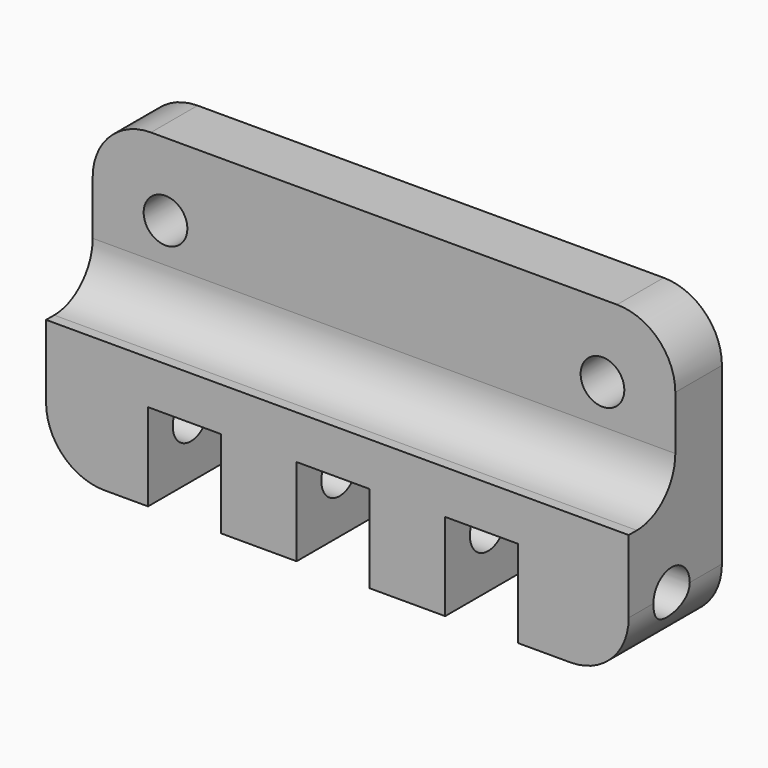
from build123d import *

# Parameters (mm, degrees)
F1_DEPTH    = 127
F2_R        = 4.7625
F3_DEPTH    = 25.4
F4_W        = 15.875
F4_H        = 19.05
F5_DEPTH    = 25.401
F6_R        = 4.953
F7_DEPTH    = 127.001
F8_T1_DEPTH = 76.2
F8_T3_DEPTH = 88.9


# Not quite as in the source:
# - a fillet or chamfer that OpenCascade refuses, or shapes differently, is made with other operations: its cross-section is extruded or revolved along the edge and cut away or added


with BuildPart() as f1:
    # F0 (on Right) → F1 (new body)
    with BuildSketch(Plane.YZ):
        with BuildLine():
            Line((0, 28.575), (0, 0))
            Line((0, 0), (25.4, 0))
            Line((25.4, 0), (25.4, 63.5))
            Line((25.4, 63.5), (12.7, 63.5))
            Line((12.7, 63.5), (12.7, 39.0525))
            ThreePointArc((12.7, 39.0525), (9.6312112999, 31.6437887001), (2.2225, 28.575))
            Line((2.2225, 28.575), (0, 28.575))
        make_face()
    extrude(amount=F1_DEPTH)

    # F2 (on face) → F3 (cut)
    with BuildSketch(Plane.XZ.offset(-12.7)):
        with Locations((111.125, 47.625)):
            Circle(F2_R)
        with Locations((15.875, 47.625)):
            Circle(F2_R)
    extrude(amount=-F3_DEPTH, mode=Mode.SUBTRACT)

    # F4 (on face) → F5 (cut, through all)
    with BuildSketch(Plane.XZ):
        with Locations((94.9325, 9.525)):
            Rectangle(F4_W, F4_H)
        with Locations((62.5475, 9.525)):
            Rectangle(F4_W, F4_H)
        with Locations((30.1625, 9.525)):
            Rectangle(F4_W, F4_H)
    extrude(amount=-F5_DEPTH, mode=Mode.SUBTRACT)

    # F6 (on face) → F7 (cut, through all)
    with BuildSketch(Plane.YZ.offset(127)):
        with Locations((11.684, 12.7)):
            Circle(F6_R)
    extrude(amount=-F7_DEPTH, mode=Mode.SUBTRACT)

    # F8: fillet of radius 12.7 on 4 edges, made by hand

    # F8_s2 → F8_t1 (cut)
    with BuildSketch(Plane.XZ.offset(-57.15)):
        with BuildLine():
            ThreePointArc((0, 50.8), (3.7197438789, 59.7802561211), (12.7, 63.5))
            Line((12.7, 63.5), (0, 63.5))
            Line((0, 63.5), (0, 50.8))
        make_face()
        with BuildLine():
            ThreePointArc((127, 50.8), (123.2802561211, 59.7802561211), (114.3, 63.5))
            Line((114.3, 63.5), (127, 63.5))
            Line((127, 63.5), (127, 50.8))
        make_face()
    extrude(amount=F8_T1_DEPTH, mode=Mode.SUBTRACT)

    # F8_s4 → F8_t3 (cut)
    with BuildSketch(Plane.XZ.offset(-57.15)):
        with BuildLine():
            ThreePointArc((0, 12.7), (3.7197438789, 3.7197438789), (12.7, 0))
            Line((12.7, 0), (0, 0))
            Line((0, 0), (0, 12.7))
        make_face()
        with BuildLine():
            ThreePointArc((127, 12.7), (123.2802561211, 3.7197438789), (114.3, 0))
            Line((114.3, 0), (127, 0))
            Line((127, 0), (127, 12.7))
        make_face()
    extrude(amount=F8_T3_DEPTH, mode=Mode.SUBTRACT)


solid = f1.part
